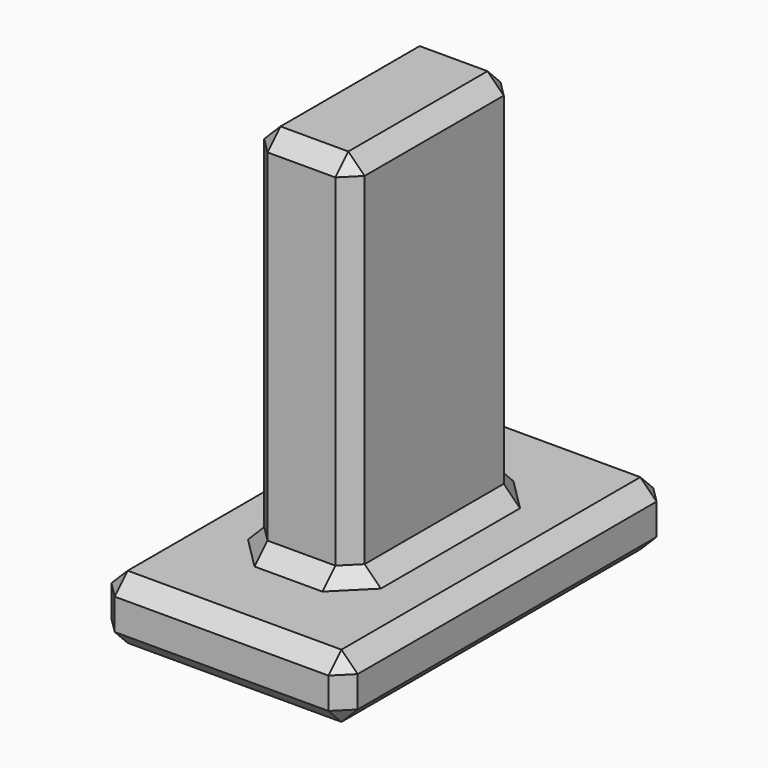
from build123d import *

# Parameters (mm, degrees)
F0_W     = 77.0167037845
F0_H     = 19.9013762176
F1_DEPTH = 63.5
F2_W     = 31.3891619444
F2_H     = 64.5581185818
F3_DEPTH = 127
F4_SIZE2 = 5.08
F4_SIZE  = 5.08


# Not quite as in the source:
# - the program builds the solid bodies; features that only make, move or delete a surface that nothing else refers to are left out


with BuildPart() as f1:
    # F0 (on Front) → F1 (new body, symmetric)
    with BuildSketch(Plane.XZ):
        Rectangle(F0_W, F0_H)
    extrude(amount=F1_DEPTH, both=True)

    # F2 (on Top) → F3 (join)
    with BuildSketch(Plane.XY):
        Rectangle(F2_W, F2_H)
    extrude(amount=F3_DEPTH)

    # F4
    f4_edges = [f1.edges().sort_by_distance(p)[0] for p in [
        (0, -32.279059, 127),
        (15.694581, -32.279059, 68.475344),
        (0, 32.279059, 127),
        (15.694581, 0, 127),
        (-15.694581, 0, 127),
        (15.694581, 32.279059, 68.475344),
        (-15.694581, 32.279059, 68.475344),
        (-15.694581, -32.279059, 68.475344),
        (15.694581, 0, 9.950688),
        (38.508352, 0, 9.950688),
        (0, -63.5, 9.950688),
        (0, 63.5, 9.950688),
        (-38.508352, 0, 9.950688),
        (0, -63.5, -9.950688),
        (-38.508352, 0, -9.950688),
        (0, 63.5, -9.950688),
        (38.508352, 0, -9.950688),
        (38.508352, 63.5, 0),
        (-38.508352, 63.5, 0),
        (38.508352, -63.5, 0),
        (-38.508352, -63.5, 0),
        (-15.694581, 0, 9.950688),
        (0, -32.279059, 9.950688),
        (0, 32.279059, 9.950688),
    ]]
    chamfer(f4_edges, length=F4_SIZE, length2=F4_SIZE2)


solid = f1.part
